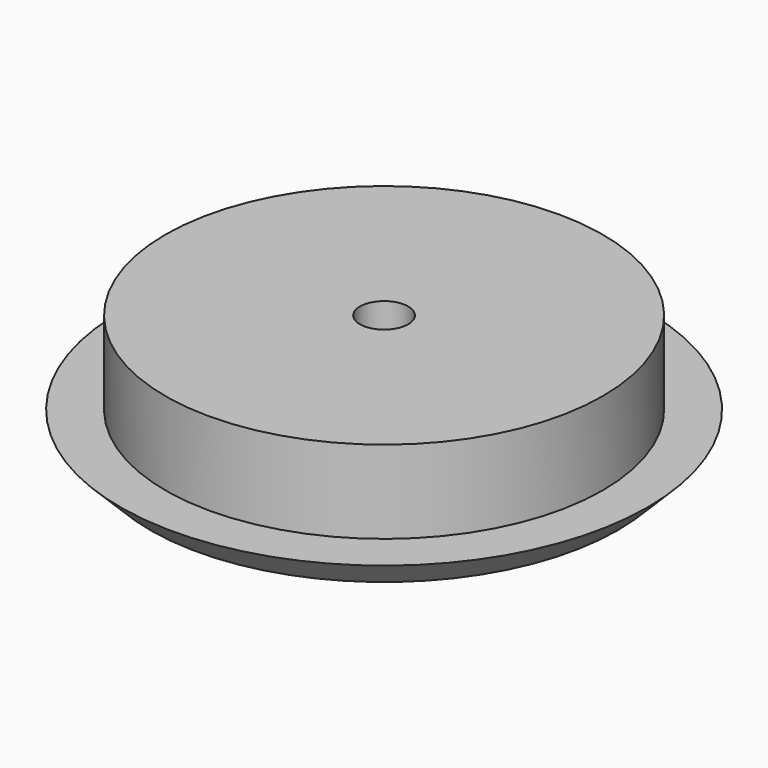
from build123d import *

# Parameters (mm, degrees)
F0_R     = 17.5
F1_DEPTH = 2
F2_R     = 14.5
F3_DEPTH = 5.5
F4_W     = 5.75
F4_H     = 5.75
F5_DEPTH = 2
F8_R     = 1.6
F9_DEPTH = 6.5
F10_SIZE = 1.99999


# Not quite as in the source:
# - a fillet or chamfer is up to 0.001 mm smaller than in the source, because OpenCascade refuses the exact size


with BuildPart() as f1:
    # F0 (on Top) → F1 (new body)
    with BuildSketch(Plane.XY):
        Circle(F0_R)
    extrude(amount=F1_DEPTH)

    # F2 (on face) → F3 (join)
    with BuildSketch(Plane.XY.offset(2)):
        Circle(F2_R)
    extrude(amount=F3_DEPTH)


with BuildPart() as f5:
    # F4 (on face) → F5 (new body)
    with BuildSketch(Plane.XY.offset(7.5)):
        with BuildLine():
            Line((-2.875, 2.875), (2.875, 2.875))
            Line((2.875, 2.875), (2.875, 14.2121207073))
            ThreePointArc((2.875, 14.2121207073), (0, 14.5), (-2.875, 14.2121207073))
            Line((-2.875, 14.2121207073), (-2.875, 2.875))
        make_face()
        Rectangle(F4_W, F4_H)
    extrude(amount=F5_DEPTH)


with BuildPart() as f5_1:
    # F6: moved
    add(f5.part.moved(Location((0, 0, -4))))


with BuildPart() as f1_1:
    add(f1.part)

    # F7: cut F5
    add(f5_1.part, mode=Mode.SUBTRACT)

    # F8 (on face) → F9 (cut)
    with BuildSketch(Plane.XY.offset(7.5)):
        Circle(F8_R)
    extrude(amount=-F9_DEPTH, mode=Mode.SUBTRACT)

    # F10 (size 2 in the source; OpenCascade refuses exactly that, so slightly less here)
    f10_edges = [f1_1.edges().sort_by_distance(p)[0] for p in [
        (-17.5, 0, 0),
    ]]
    chamfer(f10_edges, length=F10_SIZE)


solid = f1_1.part
